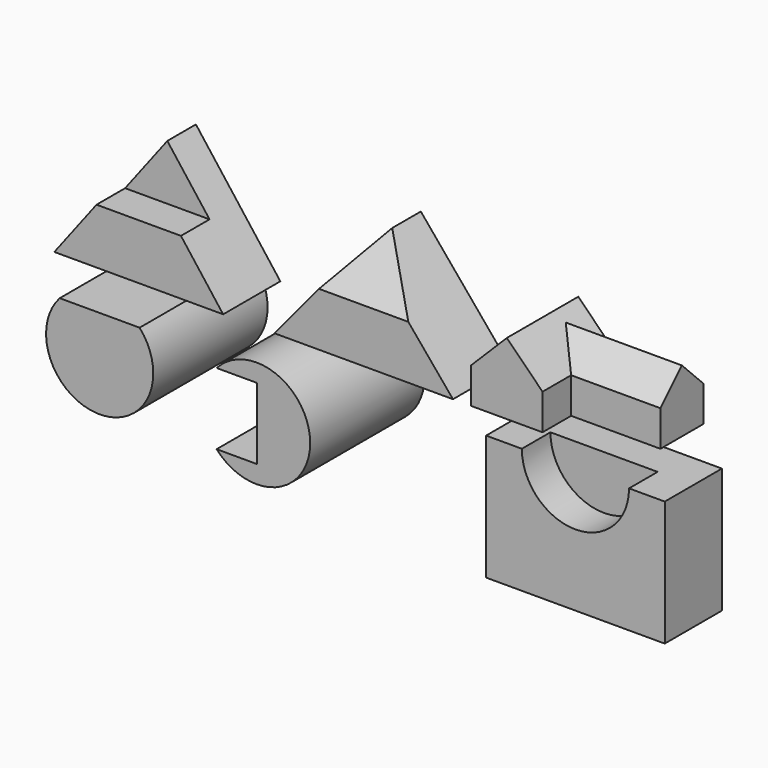
from build123d import *

# Parameters (mm, degrees)
F1_DEPTH  = 101.6
F3_DEPTH  = 50.8
F5_DEPTH  = 101.6
F10_DEPTH = 76.2
F12_DEPTH = 127
F16_R     = 76.2
F17_DEPTH = 203.2
F19_DEPTH = 101.6
F20_R     = 76.2
F21_DEPTH = 203.2
F23_DEPTH = 101.6
F24_W     = 254
F24_H     = 177.8
F25_DEPTH = 101.6
F27_DEPTH = 50.8


with BuildPart() as f1:
    # F0 (on Front) → F1 (new body)
    with BuildSketch(Plane.XZ):
        Polygon((-6.3510152444, 76.2), (-64.4574540923, 0), (175.6035333722, 0), (117.4970945244, 76.2), align=None)
        Polygon((55.57303964, 157.4063701674), (-6.3510152444, 76.2), (117.4970945244, 76.2), align=None)
    extrude(amount=-F1_DEPTH)

    # F2 (on face) → F3 (cut)
    with BuildSketch(Plane.XZ):
        Polygon((-4.4422072262, 78.7031850837), (115.5882865061, 78.7031850837), (55.57303964, 157.4063701674), align=None)
    extrude(amount=-F3_DEPTH, mode=Mode.SUBTRACT)


with BuildPart() as f5:
    # F4 (on Front) → F5 (new body)
    with BuildSketch(Plane.XZ):
        Polygon((248.3748940486, 0), (502.3748940486, 0), (375.3748940486, 152.4), align=None)
    extrude(amount=-F5_DEPTH)

    # F9 (on 3pt) → F10 (cut, symmetric)
    with BuildSketch(Plane.YZ.offset(375.3748940486)):
        Polygon((50.8, 152.4), (0, 152.4), (0, 76.2), align=None)
    extrude(amount=F10_DEPTH, both=True, mode=Mode.SUBTRACT)


with BuildPart() as f12:
    # F11 (on Front) → F12 (new body)
    with BuildSketch(Plane.XZ):
        Polygon((578.9202551112, 101.6), (528.1202551112, 50.8), (528.1202551112, 0), (629.7202551112, 0), (629.7202551112, 50.8), align=None)
    extrude(amount=-F12_DEPTH)


with BuildPart() as f15:
    # F14 (on offset) → F15 (new body, up to the next surface of F12)
    with BuildSketch(Plane.YZ.offset(756.7202551112)):
        Polygon((50.8, 0), (127, 0), (127, 50.8), (88.9, 88.9), (50.8, 50.8), align=None)
    extrude(until=Until.NEXT, target=f12.part, dir=(-1, 0, 0))


with BuildPart() as f17:
    # F16 (on Front) → F17 (new body)
    with BuildSketch(Plane.XZ):
        with Locations((0, -106.1670597964)):
            Circle(F16_R)
    extrude(amount=-F17_DEPTH)

    # F18 (on face) → F19 (cut)
    with BuildSketch(Plane.XZ):
        with BuildLine():
            ThreePointArc((56.7961266285, -55.3670597964), (0, -29.9670597964), (-56.7961266285, -55.3670597964))
            Line((-56.7961266285, -55.3670597964), (56.7961266285, -55.3670597964))
        make_face()
    extrude(amount=-F19_DEPTH, mode=Mode.SUBTRACT)


with BuildPart() as f21:
    # F20 (on Front) → F21 (new body)
    with BuildSketch(Plane.XZ):
        with Locations((223.1027185917, -121.0174635053)):
            Circle(F20_R)
    extrude(amount=-F21_DEPTH)

    # F22 (on face) → F23 (cut)
    with BuildSketch(Plane.XZ):
        with BuildLine():
            Line((223.886392215, -70.2174635053), (166.3065919632, -70.2174635053))
            ThreePointArc((166.3065919632, -70.2174635053), (146.9027185917, -121.0174635053), (166.3065919632, -171.8174635053))
            Line((166.3065919632, -171.8174635053), (223.886392215, -171.8174635053))
            Line((223.886392215, -171.8174635053), (223.886392215, -70.2174635053))
        make_face()
    extrude(amount=-F23_DEPTH, mode=Mode.SUBTRACT)


with BuildPart() as f25:
    # F24 (on Front) → F25 (new body)
    with BuildSketch(Plane.XZ):
        with Locations((676.4941598731, -119.0843340009)):
            Rectangle(F24_W, F24_H)
    extrude(amount=-F25_DEPTH)

    # F26 (on face) → F27 (cut)
    with BuildSketch(Plane.XZ):
        with BuildLine():
            ThreePointArc((600.2941598731, -30.1843340009), (676.4941598731, -106.3843340009), (752.6941598731, -30.1843340009))
            Line((752.6941598731, -30.1843340009), (600.2941598731, -30.1843340009))
        make_face()
    extrude(amount=-F27_DEPTH, mode=Mode.SUBTRACT)


solid = Compound([f1.part, f5.part, f12.part, f15.part, f17.part, f21.part, f25.part])
